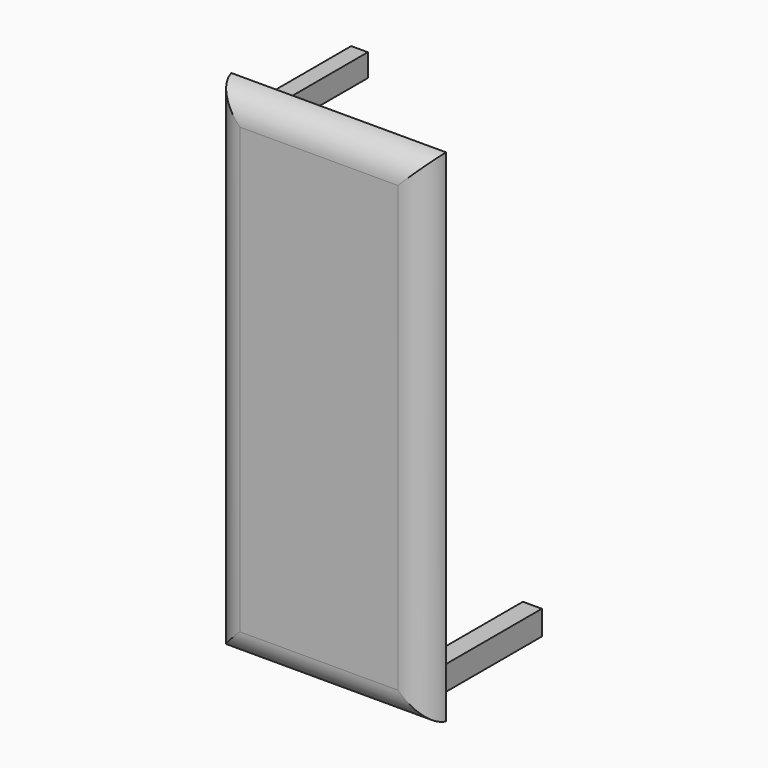
from build123d import *

# Parameters (mm, degrees)
F0_W        = 46.1472896859
F0_H        = 107.677012682
F1_DEPTH    = 5.334
F2_T1_DEPTH = 76.5470071681
F2_T3_DEPTH = 138.0767301641
F6_DEPTH    = 29.21
F8_DEPTH    = 30.226


# Not quite as in the source:
# - a fillet or chamfer that OpenCascade refuses, or shapes differently, is made with other operations: its cross-section is extruded or revolved along the edge and cut away or added
# - the program builds the solid bodies; features that only make, move or delete a surface that nothing else refers to are left out


with BuildPart() as f1:
    # F0 (on Front) → F1 (new body)
    with BuildSketch(Plane.XZ):
        with Locations((-8.118505124, 2.0296275616)):
            Rectangle(F0_W, F0_H)
    extrude(amount=F1_DEPTH)

    # F2: fillet of radius 6.1321024484 on 4 edges, made by hand

    # F2_s2 → F2_t1 (cut)
    with BuildSketch(Plane.YZ.offset(-46.392008708)):
        with BuildLine():
            ThreePointArc((0, 55.8681339025), (-3.8114922418, 53.8322375411), (-5.334, 49.7881904061))
            Line((-5.334, 49.7881904061), (-5.334, 55.8681339025))
            Line((-5.334, 55.8681339025), (0, 55.8681339025))
        make_face()
        with BuildLine():
            ThreePointArc((0, -51.8088787794), (-3.8114922418, -49.772982418), (-5.334, -45.728935283))
            Line((-5.334, -45.728935283), (-5.334, -51.8088787794))
            Line((-5.334, -51.8088787794), (0, -51.8088787794))
        make_face()
    extrude(amount=F2_T1_DEPTH, mode=Mode.SUBTRACT)

    # F2_s4 → F2_t3 (cut)
    with BuildSketch(Plane.XY.offset(-67.0087375205)):
        with BuildLine():
            ThreePointArc((-31.192149967, 0), (-29.1562536055, -3.8114922418), (-25.1122064705, -5.334))
            Line((-25.1122064705, -5.334), (-31.192149967, -5.334))
            Line((-31.192149967, -5.334), (-31.192149967, 0))
        make_face()
        with BuildLine():
            ThreePointArc((14.9551397189, 0), (12.9192433575, -3.8114922418), (8.8751962225, -5.334))
            Line((8.8751962225, -5.334), (14.9551397189, -5.334))
            Line((14.9551397189, -5.334), (14.9551397189, 0))
        make_face()
    extrude(amount=F2_T3_DEPTH, mode=Mode.SUBTRACT)

    # F5 (on Front) → F6 (join)
    with BuildSketch(Plane.XZ):
        Polygon((-25.2416264266, 49.8663634062), (-28.8135651499, 49.8663634062), (-29.4354222715, 44.9747443199), (-25.2416264266, 44.9747443199), align=None)
    extrude(amount=-F6_DEPTH)

    # F7 (on Front) → F8 (join)
    with BuildSketch(Plane.XZ):
        Polygon((11.3538028672, -49.219802022), (11.3571733236, -43.9655184746), (7.279606536, -43.9655184746), (7.279606536, -49.219802022), align=None)
    extrude(amount=-F8_DEPTH)


solid = f1.part
